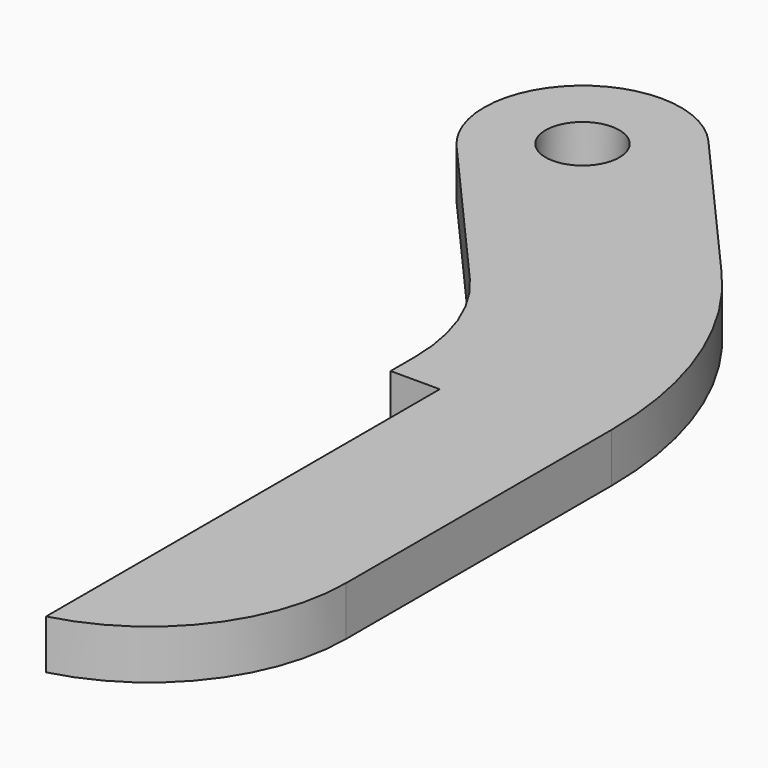
from build123d import *

# Parameters (mm, degrees)
F0_R        = 4.7625
F1_DEPTH    = 6.35
F2_T1_DEPTH = 6.35
F2_T3_DEPTH = 129.3172212421
F3_R        = 50.8


# Not quite as in the source:
# - a fillet or chamfer that OpenCascade refuses, or shapes differently, is made with other operations: its cross-section is extruded or revolved along the edge and cut away or added


with BuildPart() as f1:
    # F0 (on Top) → F1 (new body)
    with BuildSketch(Plane.XY):
        with BuildLine():
            Line((25.4, -63.5), (25.4, 23.0659139254))
            Line((25.4, 23.0659139254), (-6.3346226919, 59.1827919466))
            ThreePointArc((-6.3346226919, 59.1827919466), (-24.2577919466, 60.3403773081), (-25.4153773081, 42.4172080534))
            Line((-25.4153773081, 42.4172080534), (0, 13.4922042489))
            Line((0, 13.4922042489), (0, 0))
            Line((0, 0), (6.35, 0))
            Line((6.35, 0), (6.35, -63.5))
            Line((6.35, -63.5), (25.4, -63.5))
        make_face()
        with Locations((-15.875, 50.8)):
            Circle(F0_R, mode=Mode.SUBTRACT)
    extrude(amount=F1_DEPTH)

    # F2: fillet of radius 25.4 on 2 edges, made by hand

    # F2_s2 → F2_t1 (join)
    with BuildSketch(Plane.XY):
        with BuildLine():
            ThreePointArc((-6.3192453838, 20.6840784656), (-1.6322574983, 12.8769775006), (0, 3.9184945725))
            Line((0, 3.9184945725), (0, 13.4922042489))
            Line((0, 13.4922042489), (-6.3192453838, 20.6840784656))
        make_face()
    extrude(amount=F2_T1_DEPTH)

    # F2_s4 → F2_t3 (cut)
    with BuildSketch(Plane.XY.offset(-61.483610621)):
        with BuildLine():
            ThreePointArc((6.35, -63.5), (20.0804631421, -54.4608156183), (25.4, -38.9065557516))
            Line((25.4, -38.9065557516), (25.4, -63.5))
            Line((25.4, -63.5), (6.35, -63.5))
        make_face()
    extrude(amount=F2_T3_DEPTH, mode=Mode.SUBTRACT)

    # F3
    f3_edges = [f1.edges().sort_by_distance(p)[0] for p in [
        (25.4, 23.065914, 3.175),
    ]]
    fillet(f3_edges, radius=F3_R)


solid = f1.part
